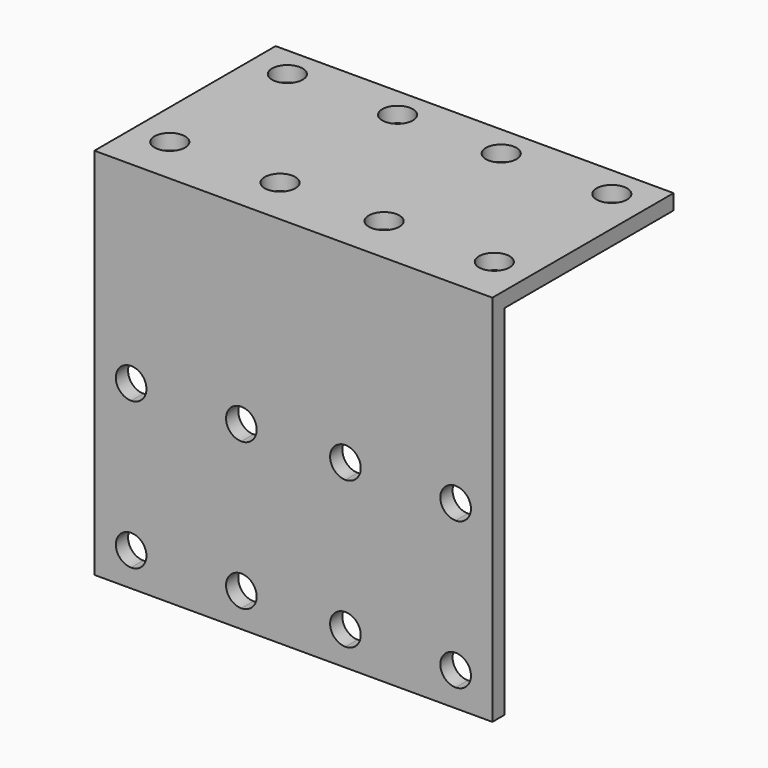
from build123d import *

# Parameters (mm, degrees)
F0_W     = 2.5
F0_H     = 58.5
F1_DEPTH = 32.5
F3_DEPTH = 5
F4_R     = 2.5
F5_DEPTH = 5


with BuildPart() as f1:
    # F0 (on Right) → F1 (new body, symmetric)
    with BuildSketch(Plane.YZ):
        Polygon((0, 2.5), (0, 0), (2.5, 0), (37, 0), (37, 2.5), align=None)
        with Locations((1.25, -29.25)):
            Rectangle(F0_W, F0_H)
    extrude(amount=F1_DEPTH, both=True)

    # F2 (on Front) → F3 (cut, symmetric)
    with BuildSketch(Plane.XZ):
        with BuildLine():
            Line((-26.5, -31.5), (-26.5, -26.5))
            ThreePointArc((-26.5, -26.5), (-29, -29), (-26.5, -31.5))
        make_face()
        with BuildLine():
            ThreePointArc((-26.5, -31.5), (-24.732233047, -30.767766953), (-24, -29))
            ThreePointArc((-24, -29), (-24.732233047, -27.232233047), (-26.5, -26.5))
            Line((-26.5, -26.5), (-26.5, -31.5))
        make_face()
        with BuildLine():
            Line((-8.5, -31.5), (-8.5, -26.5))
            ThreePointArc((-8.5, -26.5), (-11, -29), (-8.5, -31.5))
        make_face()
        with BuildLine():
            ThreePointArc((-8.5, -31.5), (-6.732233047, -30.767766953), (-6, -29))
            ThreePointArc((-6, -29), (-6.732233047, -27.232233047), (-8.5, -26.5))
            Line((-8.5, -26.5), (-8.5, -31.5))
        make_face()
        with BuildLine():
            Line((8.5, -31.5), (8.5, -26.5))
            ThreePointArc((8.5, -26.5), (6, -29), (8.5, -31.5))
        make_face()
        with BuildLine():
            ThreePointArc((8.5, -31.5), (10.267766953, -30.767766953), (11, -29))
            ThreePointArc((11, -29), (10.267766953, -27.232233047), (8.5, -26.5))
            Line((8.5, -26.5), (8.5, -31.5))
        make_face()
        with BuildLine():
            Line((26.5, -31.5), (26.5, -26.5))
            ThreePointArc((26.5, -26.5), (24, -29), (26.5, -31.5))
        make_face()
        with BuildLine():
            ThreePointArc((26.5, -31.5), (28.267766953, -30.767766953), (29, -29))
            ThreePointArc((29, -29), (28.267766953, -27.232233047), (26.5, -26.5))
            Line((26.5, -26.5), (26.5, -31.5))
        make_face()
        with BuildLine():
            Line((-26.5, -55.5), (-26.5, -50.5))
            ThreePointArc((-26.5, -50.5), (-29, -53), (-26.5, -55.5))
        make_face()
        with BuildLine():
            ThreePointArc((-24, -53), (-24.732233047, -51.232233047), (-26.5, -50.5))
            Line((-26.5, -50.5), (-26.5, -55.5))
            ThreePointArc((-26.5, -55.5), (-24.732233047, -54.767766953), (-24, -53))
        make_face()
        with BuildLine():
            ThreePointArc((-6, -53), (-6.732233047, -51.232233047), (-8.5, -50.5))
            Line((-8.5, -50.5), (-8.5, -55.5))
            ThreePointArc((-8.5, -55.5), (-6.732233047, -54.767766953), (-6, -53))
        make_face()
        with BuildLine():
            Line((-8.5, -55.5), (-8.5, -50.5))
            ThreePointArc((-8.5, -50.5), (-11, -53), (-8.5, -55.5))
        make_face()
        with BuildLine():
            ThreePointArc((11, -53), (10.267766953, -51.232233047), (8.5, -50.5))
            Line((8.5, -50.5), (8.5, -55.5))
            ThreePointArc((8.5, -55.5), (10.267766953, -54.767766953), (11, -53))
        make_face()
        with BuildLine():
            Line((8.5, -55.5), (8.5, -50.5))
            ThreePointArc((8.5, -50.5), (6, -53), (8.5, -55.5))
        make_face()
        with BuildLine():
            ThreePointArc((29, -53), (28.267766953, -51.232233047), (26.5, -50.5))
            Line((26.5, -50.5), (26.5, -55.5))
            ThreePointArc((26.5, -55.5), (28.267766953, -54.767766953), (29, -53))
        make_face()
        with BuildLine():
            Line((26.5, -55.5), (26.5, -50.5))
            ThreePointArc((26.5, -50.5), (24, -53), (26.5, -55.5))
        make_face()
    extrude(amount=F3_DEPTH, both=True, mode=Mode.SUBTRACT)

    # F4 (on face) → F5 (cut, symmetric)
    with BuildSketch(Plane.XY.offset(2.5)):
        with Locations((-26.5, 7.894)):
            Circle(F4_R)
        with Locations((-26.5, 31.894)):
            Circle(F4_R)
        with Locations((-8.5, 31.894)):
            Circle(F4_R)
        with Locations((-8.5, 7.894)):
            Circle(F4_R)
        with Locations((8.5, 7.894)):
            Circle(F4_R)
        with Locations((8.5, 31.8015553057)):
            Circle(F4_R)
        with Locations((26.5, 31.894)):
            Circle(F4_R)
        with Locations((26.5, 7.894)):
            Circle(F4_R)
    extrude(amount=F5_DEPTH, both=True, mode=Mode.SUBTRACT)


solid = f1.part
